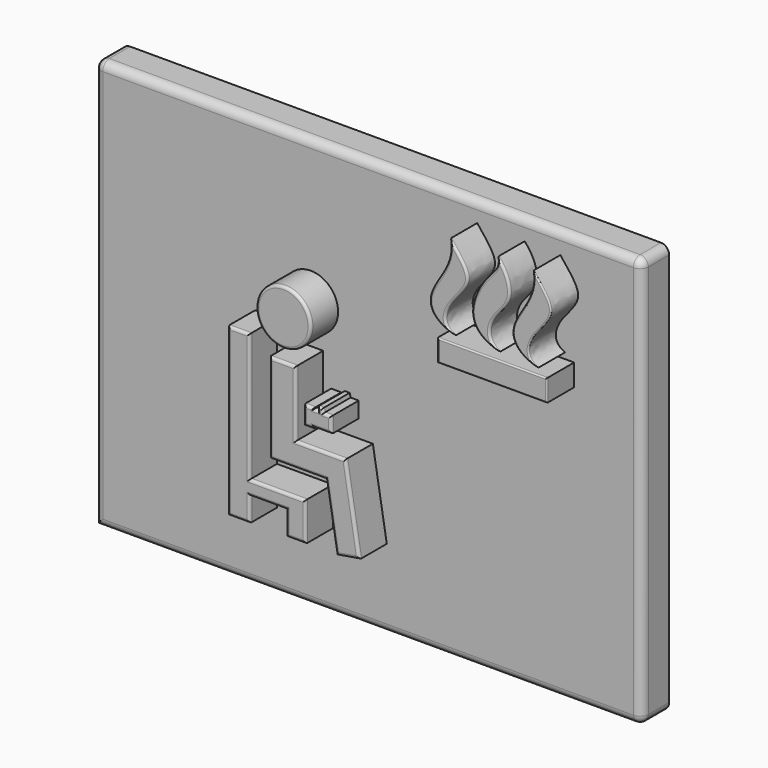
from build123d import *

# Parameters (mm, degrees)
F0_W          = 50.8
F0_H          = 38.1
F1_DEPTH      = 3.175
F2_R          = 2.54
F3_DEPTH      = 3.175
F4_DEPTH      = 3.175
F5_R          = 0.254
F6_W          = 10.16
F6_H          = 2.032
F7_DEPTH      = 3.175
F8_R          = 0.127
F9_R          = 0.2032
F10_R         = 0.762
F11_T1_DEPTH  = 4.318
F11_S5_W      = 0.762
F11_S5_H      = 0.762
F11_T6_DEPTH  = 0.762
F11_S11_W     = 0.762
F11_S11_H     = 0.762
F11_T12_DEPTH = 0.762
F11_S17_W     = 0.762
F11_S17_H     = 0.762
F11_T18_DEPTH = 0.762


# Not quite as in the source:
# - a fillet or chamfer that OpenCascade refuses, or shapes differently, is made with other operations: its cross-section is extruded or revolved along the edge and cut away or added
# - a feature names something its author has since deleted; it is built from what else it names


with BuildPart() as f1:
    # F0 (on Front) → F1 (new body)
    with BuildSketch(Plane.XZ):
        with Locations((6.6340767503, -14.1872374833)):
            Rectangle(F0_W, F0_H)
    extrude(amount=F1_DEPTH)

    # F2 (on face) → F3 (join)
    with BuildSketch(Plane.XZ.offset(3.175)):
        Polygon((2.4591459114, -12.0548624545), (0, -12.0548624545), (0, -20.3714100644), (5.2313286033, -20.3714100644), (6.2150064078, -26.2734768912), (8.361211744, -25.9157760018), (7.0681710327, -18.1575317339), (2.4591459114, -18.1575317339), align=None)
        Polygon((-1.833265469, -22.6964680478), (-1.833265469, -12.0548624545), (-1.833265469, -10.7978451997), (-3.8587087147, -10.7978451997), (-3.8587087147, -26.2734768912), (-1.833265469, -26.2734768912), (-1.833265469, -24.0378165618), (1.5648935842, -24.0378165618), (1.5648935842, -26.2734768912), (3.353398588, -26.2734768912), (3.353398588, -22.6964680478), align=None)
        with Locations((1.3011579867, -8.4271756932)):
            Circle(F2_R)
    extrude(amount=F3_DEPTH)

    # F2 (on face) → F4 (join)
    with BuildSketch(Plane.XZ.offset(3.175)):
        with Locations((1.3011579867, -8.4271756932)):
            Circle(F2_R)
        Polygon((2.4591459114, -12.0548624545), (0, -12.0548624545), (0, -20.3714100644), (5.2313286033, -20.3714100644), (6.2150064078, -26.2734768912), (8.361211744, -25.9157760018), (7.0681710327, -18.1575317339), (2.4591459114, -18.1575317339), align=None)
        Polygon((-1.833265469, -22.6964680478), (-1.833265469, -12.0548624545), (-1.833265469, -10.7978451997), (-3.8587087147, -10.7978451997), (-3.8587087147, -26.2734768912), (-1.833265469, -26.2734768912), (-1.833265469, -24.0378165618), (1.5648935842, -24.0378165618), (1.5648935842, -26.2734768912), (3.353398588, -26.2734768912), (3.353398588, -22.6964680478), align=None)
        Polygon((4.1369330138, -14.9092301726), (3.1979684718, -14.9092301726), (3.1979684718, -16.6530236602), (4.1369330138, -16.6530236602), (4.1369330138, -16.5201351047), (4.1369330138, -14.9977691472), align=None)
        Polygon((4.4626258314, -14.9977691472), (4.1369330138, -14.9977691472), (4.1369330138, -16.5201351047), (5.7552675717, -16.5201351047), (5.7552675717, -15.0536596775), (5.0036055036, -15.0536596775), (4.9177779964, -14.6928746253), (4.4626258314, -14.6928746253), align=None)
    extrude(amount=F4_DEPTH)

    # F5
    f5_edges = [f1.edges().sort_by_distance(p)[0] for p in [
        (-3.858709, -6.35, -18.535661),
        (-2.845987, -6.35, -10.797845),
        (-1.833265, -6.35, -16.747157),
        (-1.238842, -6.35, -8.427176),
        (0, -6.35, -16.213136),
        (1.229573, -6.35, -12.054862),
        (2.459146, -6.35, -15.106197),
        (4.763658, -6.35, -18.157532),
        (7.714691, -6.35, -22.036654),
        (7.288109, -6.35, -26.094626),
        (5.723168, -6.35, -23.322443),
        (2.615664, -6.35, -20.37141),
        (-2.845987, -6.35, -26.273477),
        (-1.833265, -6.35, -25.155647),
        (-0.134186, -6.35, -24.037817),
        (0.760067, -6.35, -22.696468),
        (1.564894, -6.35, -25.155647),
        (2.459146, -6.35, -26.273477),
        (3.353399, -6.35, -24.484972),
        (4.9461, -6.35, -16.520135),
        (3.667451, -6.35, -16.653024),
        (4.136933, -6.35, -16.586579),
        (5.755268, -6.35, -15.786897),
        (5.379437, -6.35, -15.05366),
        (4.960692, -6.35, -14.873267),
        (4.690202, -6.35, -14.692875),
        (4.462626, -6.35, -14.845322),
        (4.299779, -6.35, -14.997769),
        (4.136933, -6.35, -14.9535),
        (3.667451, -6.35, -14.90923),
        (3.197968, -6.35, -15.781127),
    ]]
    fillet(f5_edges, radius=F5_R)

    # F6 (on face) → F7 (join)
    with BuildSketch(Plane.XZ.offset(3.175)):
        with Locations((20.6759455931, -6.4530780602)):
            Rectangle(F6_W, F6_H)
        with BuildLine():
            add(Edge.make_bspline(
                [(24.9169189483, -4.8799356446), (23.3313957528, -4.4876471111), (21.8683446082, -2.7486966543), (24.0372652567, -0.0026418092), (24.6774328786, 1.8384480061), (24.4763102382, 2.9274572153)],
                knots=[0, 0, 0, 0, 0.3409433415, 0.6695367123, 1, 1, 1, 1], degree=3))
            add(Edge.make_bspline(
                [(24.9169189483, -4.8799356446), (23.8370091624, -4.4573652119), (24.014534853, -2.4017894935), (27.1180160286, -0.0161511815), (25.3185529396, 1.8161626677), (24.4763102382, 2.9274572153)],
                knots=[0, 0, 0, 0, 0.2930700859, 0.6424542626, 1, 1, 1, 1], degree=3))
        make_face()
        with BuildLine():
            add(Edge.make_bspline(
                [(21.3134847581, -4.7694058158), (19.6643419971, -4.3613765942), (18.0534780672, -2.5461416843), (20.065856741, 1.1675050618), (21.3361559436, 2.0479429176), (21.1639329791, 2.9804704245)],
                knots=[0, 0, 0, 0, 0.3546237893, 0.7170215796, 1, 1, 1, 1], degree=3))
            add(Edge.make_bspline(
                [(21.3134847581, -4.7694058158), (20.2167103489, -4.186536189), (20.4242312758, -2.0796513875), (22.834879683, -0.4029217906), (22.1232692814, 1.9297199332), (21.1639329791, 2.9804704245)],
                knots=[0, 0, 0, 0, 0.3135886137, 0.6343920972, 1, 1, 1, 1], degree=3))
        make_face()
        with BuildLine():
            add(Edge.make_bspline(
                [(17.1978485734, -4.7740393784), (15.6123253779, -4.3817508449), (14.1492742333, -2.6428003882), (16.3181948818, 0.103254457), (16.9583625037, 1.9443442722), (16.7572398633, 3.0333534814)],
                knots=[0, 0, 0, 0, 0.3409433415, 0.6695367123, 1, 1, 1, 1], degree=3))
            add(Edge.make_bspline(
                [(17.1978485734, -4.7740393784), (16.1179387874, -4.3514689457), (16.2954644781, -2.2958932273), (19.3989456537, 0.0897450846), (17.5994825647, 1.9220589338), (16.7572398633, 3.0333534814)],
                knots=[0, 0, 0, 0, 0.2930700859, 0.6424542626, 1, 1, 1, 1], degree=3))
        make_face()
    extrude(amount=F7_DEPTH)

    # F8
    f8_edges = [f1.edges().sort_by_distance(p)[0] for p in [
        (22.97696, -6.35, -1.4519),
        (25.58246, -6.35, -1.081727),
        (25.755946, -6.35, -6.453078),
        (20.675946, -6.35, -5.437078),
        (20.675946, -6.35, -7.469078),
        (15.595946, -6.35, -6.453078),
    ]]
    fillet(f8_edges, radius=F8_R)

    # F9
    f9_edges = [f1.edges().sort_by_distance(p)[0] for p in [
        (21.74311, -6.35, -1.041175),
        (18.979674, -6.35, -1.241282),
        (17.86339, -6.35, -0.975831),
        (15.25789, -6.35, -1.346004),
        (23.252255, -6.35, -1.216465),
        (25.58246, -6.223, -1.081727),
    ]]
    fillet(f9_edges, radius=F9_R)

    # F10
    f10_edges = [f1.edges().sort_by_distance(p)[0] for p in [
        (32.034077, -3.175, -14.187237),
        (6.634077, -3.175, -33.237237),
        (6.634077, -3.175, 4.862763),
        (-18.765923, -3.175, -14.187237),
    ]]
    fillet(f10_edges, radius=F10_R)

    # F11: fillet of radius 0.762 on 3 edges, made by hand

    # F11_s2 → F11_t1 (cut)
    with BuildSketch(Plane.XZ.offset(-1.905)):
        with BuildLine():
            ThreePointArc((32.0340767503, 4.1007625167), (31.8108921175, 4.639577884), (31.2720767503, 4.8627625167))
            Line((31.2720767503, 4.8627625167), (32.0340767503, 4.8627625167))
            Line((32.0340767503, 4.8627625167), (32.0340767503, 4.1007625167))
        make_face()
        with BuildLine():
            ThreePointArc((-18.0039232497, 4.8627625167), (-18.542738617, 4.639577884), (-18.7659232497, 4.1007625167))
            Line((-18.7659232497, 4.1007625167), (-18.7659232497, 4.8627625167))
            Line((-18.7659232497, 4.8627625167), (-18.0039232497, 4.8627625167))
        make_face()
        with BuildLine():
            ThreePointArc((32.0340767503, -32.4752374833), (31.8108921175, -33.0140528505), (31.2720767503, -33.2372374833))
            Line((31.2720767503, -33.2372374833), (32.0340767503, -33.2372374833))
            Line((32.0340767503, -33.2372374833), (32.0340767503, -32.4752374833))
        make_face()
    extrude(amount=F11_T1_DEPTH, mode=Mode.SUBTRACT)


with BuildPart() as f11_tool4:
    # F11_s5 → F11_t6 (new body)
    with BuildSketch(Plane.YZ.offset(31.2720767503)):
        with Locations((-2.794, -32.8562374833)):
            Rectangle(F11_S5_W, F11_S5_H)
    extrude(amount=F11_T6_DEPTH)

    # F11_s7 → F11_t8 (revolve, cut)
    with BuildSketch(Plane(origin=(31.2720767503, -2.413, -32.4752374833), x_dir=(0, 0.7071067812, 0.7071067812), z_dir=(0, 0.7071067812, -0.7071067812))):
        with BuildLine():
            ThreePointArc((0, -0.762), (0.762, 0), (0, 0.762))
            Line((0, 0.762), (0, -0.762))
        make_face()
    revolve(axis=Axis((31.2720767503, -2.413, -32.4752374833), (1, 0, 0)), mode=Mode.SUBTRACT)


with BuildPart() as f1_1:
    add(f1.part)

    # F11_t3: cut F11_tool4
    add(f11_tool4.part, mode=Mode.SUBTRACT)


with BuildPart() as f11_tool10:
    # F11_s11 → F11_t12 (new body)
    with BuildSketch(Plane.XY.offset(4.1007625167)):
        with Locations((-18.3849232497, -2.794)):
            Rectangle(F11_S11_W, F11_S11_H)
    extrude(amount=F11_T12_DEPTH)

    # F11_s13 → F11_t14 (revolve, cut)
    with BuildSketch(Plane(origin=(-18.0039232497, -2.413, 4.1007625167), x_dir=(0.7071067812, 0.7071067812, 0), z_dir=(0.7071067812, -0.7071067812, 0))):
        with BuildLine():
            ThreePointArc((0, -0.762), (0.762, 0), (0, 0.762))
            Line((0, 0.762), (0, -0.762))
        make_face()
    revolve(axis=Axis((-18.0039232497, -2.413, 4.1007625167), (0, 0, 1)), mode=Mode.SUBTRACT)


with BuildPart() as f1_2:
    add(f1_1.part)

    # F11_t9: cut F11_tool10
    add(f11_tool10.part, mode=Mode.SUBTRACT)


with BuildPart() as f11_tool16:
    # F11_s17 → F11_t18 (new body)
    with BuildSketch(Plane.YZ.offset(31.2720767503)):
        with Locations((-2.794, 4.4817625167)):
            Rectangle(F11_S17_W, F11_S17_H)
    extrude(amount=F11_T18_DEPTH)

    # F11_s19 → F11_t20 (revolve, cut)
    with BuildSketch(Plane(origin=(31.2720767503, -2.413, 4.1007625167), x_dir=(0, 0.7071067812, -0.7071067812), z_dir=(0, -0.7071067812, -0.7071067812))):
        with BuildLine():
            ThreePointArc((0, -0.762), (0.762, 0), (0, 0.762))
            Line((0, 0.762), (0, -0.762))
        make_face()
    revolve(axis=Axis((31.2720767503, -2.413, 4.1007625167), (1, 0, 0)), mode=Mode.SUBTRACT)


with BuildPart() as f1_3:
    add(f1_2.part)

    # F11_t15: cut F11_tool16
    add(f11_tool16.part, mode=Mode.SUBTRACT)


solid = f1_3.part
